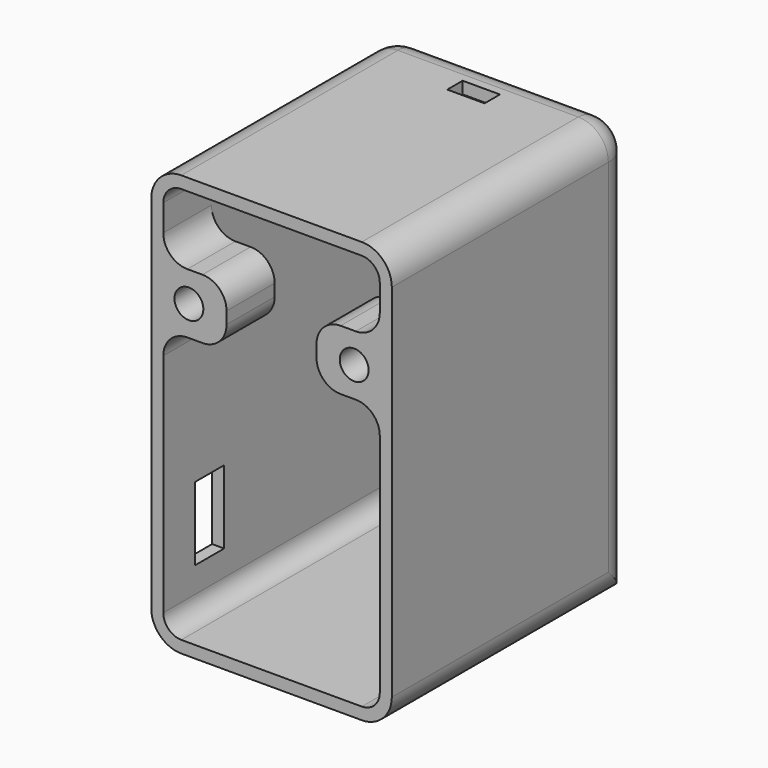
from build123d import *

# Parameters (mm, degrees)
F0_W      = 50.8
F0_H      = 88.9
F1_DEPTH  = 63.5
F2_R      = 6.35
F3_T      = -2.54
F4_W      = 15.9004
F4_H      = 12.7
F4_R      = 3.048
F5_DEPTH  = 12.7
F6_R      = 5.08
F7_W      = 7.874
F7_H      = 4.064
F8_DEPTH  = 25.4
F9_W      = 1.27
F9_H      = 25.4
F10_DEPTH = 11.43
F11_W     = 16.129
F11_H     = 16.0528
F12_DEPTH = 13.843
F11_W_2   = 18.669
F11_H_2   = 18.5928
F13_DEPTH = 13.843
F14_W     = 3.7612880599
F14_H     = 9.271
F15_DEPTH = 13.843
F16_W     = 18.669
F16_H     = 18.5928
F17_DEPTH = 1.27
F18_W     = 7.6708
F18_H     = 15.494
F19_DEPTH = 25.4


with BuildPart() as f1:
    # F0 (on Front) → F1 (new body)
    with BuildSketch(Plane.XZ):
        Rectangle(F0_W, F0_H)
    extrude(amount=F1_DEPTH)

    # F2
    f2_edges = [f1.edges().sort_by_distance(p)[0] for p in [
        (25.4, -31.75, 44.45),
        (-25.4, -31.75, 44.45),
        (0, 0, 44.45),
        (25.4, -31.75, -44.45),
        (-25.4, -31.75, -44.45),
        (25.4, 0, 0),
        (-25.4, 0, 0),
    ]]
    fillet(f2_edges, radius=F2_R)

    # F3
    f3_openings = [f1.faces().sort_by_distance(p)[0] for p in [
        (0, -63.5, 0),
    ]]
    offset(amount=F3_T, openings=f3_openings)

    # F4 (on face) → F5 (join)
    with BuildSketch(Plane.XZ.offset(63.5)):
        with Locations((-17.4498, 21.082)):
            Rectangle(F4_W, F4_H)
        with Locations((-17.4498, 21.082)):
            Circle(F4_R, mode=Mode.SUBTRACT)
        with Locations((17.4498, 21.082)):
            Rectangle(F4_W, F4_H)
        with Locations((17.4498, 21.082)):
            Circle(F4_R, mode=Mode.SUBTRACT)
    extrude(amount=-F5_DEPTH)

    # F6
    f6_edges = [f1.edges().sort_by_distance(p)[0] for p in [
        (-9.4996, -57.15, 27.432),
        (-9.4996, -57.15, 14.732),
        (9.4996, -57.15, 14.732),
        (9.4996, -57.15, 27.432),
        (-22.86, -57.15, 27.432),
        (22.86, -57.15, 27.432),
        (-22.86, -57.15, 14.732),
        (22.86, -57.15, 14.732),
    ]]
    fillet(f6_edges, radius=F6_R)

    # F7 (on face) → F8 (cut)
    with BuildSketch(Plane.XY.offset(44.45)):
        with Locations((0, -10.16)):
            Rectangle(F7_W, F7_H)
    extrude(amount=-F8_DEPTH, mode=Mode.SUBTRACT)

    # F9 (on face) → F10 (join)
    with BuildSketch(Plane.XZ.offset(2.54)):
        with Locations((-9.525, 25.4)):
            Rectangle(F9_W, F9_H)
        with Locations((9.525, 25.4)):
            Rectangle(F9_W, F9_H)
    extrude(amount=F10_DEPTH)

    # F11 (on face) → F12 (cut)
    with BuildSketch(Plane(origin=(0, 0, 0), x_dir=(-1, 0, 0), z_dir=(0, 1, 0))):
        with Locations((0, -35.1536)):
            Rectangle(F11_W, F11_H)
    extrude(amount=-F12_DEPTH, mode=Mode.SUBTRACT)

    # F11 (on face) → F13 (join)
    with BuildSketch(Plane(origin=(0, 0, 0), x_dir=(-1, 0, 0), z_dir=(0, 1, 0))):
        with Locations((0, -35.1536)):
            Rectangle(F11_W_2, F11_H_2)
        with Locations((0, -35.1536)):
            Rectangle(F11_W, F11_H, mode=Mode.SUBTRACT)
    extrude(amount=-F13_DEPTH)

    # F14 (on face) → F15 (cut)
    with BuildSketch(Plane(origin=(0, 0, 0), x_dir=(-1, 0, 0), z_dir=(0, 1, 0))):
        with Locations((-7.45385597, -35.1536)):
            Rectangle(F14_W, F14_H)
    extrude(amount=-F15_DEPTH, mode=Mode.SUBTRACT)

    # F16 (on face) → F17 (join)
    with BuildSketch(Plane.XZ.offset(13.843)):
        with Locations((0, -35.1536)):
            Rectangle(F16_W, F16_H)
    extrude(amount=F17_DEPTH)

    # F18 (on face) → F19 (cut)
    with BuildSketch(Plane(origin=(-25.4, 0, 0), x_dir=(0, -1, 0), z_dir=(-1, 0, 0))):
        with Locations((51.2709531141, -24.9448278919)):
            Rectangle(F18_W, F18_H)
    extrude(amount=-F19_DEPTH, mode=Mode.SUBTRACT)


solid = f1.part
